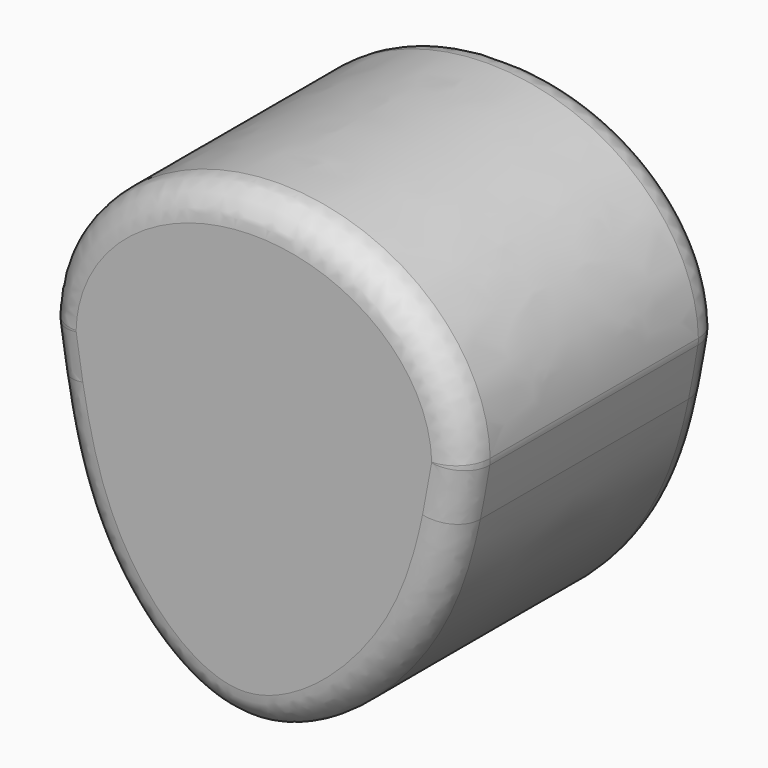
from build123d import *

# Parameters (mm, degrees)
F1_DEPTH = 50.8
F3_F1_R  = 5.08
F3_F2_R  = 5.08
F3_F3_R  = 5.08
F3_F4_R  = 5.08


with BuildPart() as f1:
    # F0 (on Front) → F1 (new body)
    with BuildSketch(Plane.XZ):
        with BuildLine():
            add(Edge.make_bspline(
                [(26.8634640441, 30.0725474095), (27.4503774573, 32.8547975525), (27.9298393949, 35.6489431931), (28.4093022346, 38.4430885315)],
                knots=[0.9262660757, 0.9262660757, 0.9262660757, 0.9262660757, 1, 1, 1, 1], degree=3))
            add(Edge.make_bspline(
                [(28.4093022346, 38.4430885315), (28.4093022346, 66.056851956), (-4.4455230236, 66.056851956), (-37.3003482819, 66.056851956), (-37.3003482819, 38.4430885315)],
                knots=[0, 0, 0, 1.5707963268, 1.5707963268, 3.1415926536, 3.1415926536, 3.1415926536], degree=2, weights=[1, 0.7071067812, 1, 0.7071067812, 1]))
            add(Edge.make_bspline(
                [(-37.3003482819, 38.4430885315), (-36.939333387, 36.041498013), (-36.5783185118, 33.6399074922), (-36.1667983256, 31.2521979805)],
                knots=[0, 0, 0, 0, 0.0600642843, 0.0600642843, 0.0600642843, 0.0600642843], degree=3))
            add(Edge.make_bspline(
                [(-36.1667983256, 31.2521979805), (-7.0407045556, -59.5095977908), (26.8634640441, 30.0725474095)],
                knots=[3.405039124, 3.405039124, 3.405039124, 5.9752105426, 5.9752105426, 5.9752105426], degree=2, weights=[1, 0.2818393326, 1]))
        make_face()
        with BuildLine():
            add(Edge.make_bspline(
                [(-36.1667983256, 31.2521979805), (-34.8445259273, 23.5801505614), (-30.6813709026, 6.5799650339), (-6.2447021875, -15.5619977157), (20.5872658458, 7.4633058375), (25.4857013307, 23.5412935316), (26.8634640441, 30.0725474095)],
                knots=[0.0600642843, 0.0600642843, 0.0600642843, 0.0600642843, 0.2530593012, 0.4958547101, 0.7531777644, 0.9262660757, 0.9262660757, 0.9262660757, 0.9262660757], degree=3))
            add(Edge.make_bspline(
                [(-36.1667983256, 31.2521979805), (-7.0407045556, -59.5095977908), (26.8634640441, 30.0725474095)],
                knots=[3.405039124, 3.405039124, 3.405039124, 5.9752105426, 5.9752105426, 5.9752105426], degree=2, weights=[1, 0.2818393326, 1]))
        make_face()
    extrude(amount=F1_DEPTH)

    # F3: fillet of radius 5.08 on 6 edges, made by hand

    # F3_f1
    f3_f1_edges = [f1.edges().sort_by_distance(p)[0] for p in [
        (28.4093022346, -25.4, 38.4430885315),
    ]]
    fillet(f3_f1_edges, radius=F3_F1_R)

    # F3_f2
    f3_f2_edges = [f1.edges().sort_by_distance(p)[0] for p in [
        (-37.3003482819, -25.4, 38.4430885315),
    ]]
    fillet(f3_f2_edges, radius=F3_F2_R)

    # F3_f3
    f3_f3_edges = [f1.edges().sort_by_distance(p)[0] for p in [
        (-4.4832090892, 0, 66.05683379),
    ]]
    fillet(f3_f3_edges, radius=F3_F3_R)

    # F3_f4
    f3_f4_edges = [f1.edges().sort_by_distance(p)[0] for p in [
        (-4.4832090892, -50.8, 66.05683379),
    ]]
    fillet(f3_f4_edges, radius=F3_F4_R)


solid = f1.part
